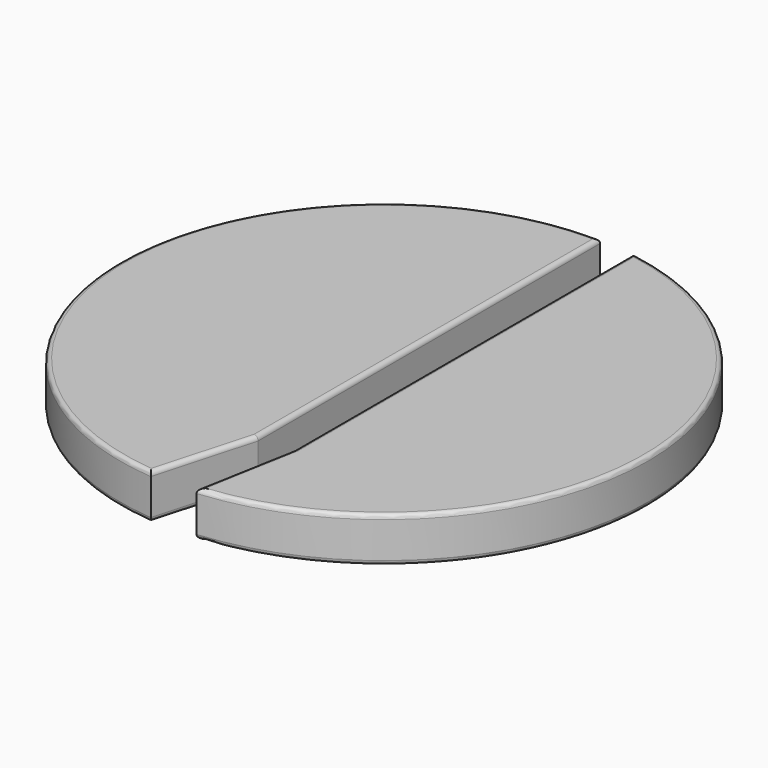
from build123d import *

# Parameters (mm, degrees)
F1_DEPTH      = 3.78
F2_T4_DEPTH   = 40.3204423055
F2_T9_DEPTH   = 12.9439682299
F2_T14_DEPTH  = 12.9439682299
F2_T19_DEPTH  = 40.3204423055
F2_T22_ANGLE  = 177.5138742153
F2_T24_ANGLE  = 177.5138742153
F2_T29_DEPTH  = 40.3204423055
F2_T33_DEPTH  = 12.9439682299
F2_T40_DEPTH  = 40.3204423055
F2_T44_DEPTH  = 12.9439682299
F2_2_T1_DEPTH = 38.6518237684
F2_2_T3_DEPTH = 11.2008796601
F2_2_T6_ANGLE = 180.8453878552
F2_2_T8_ANGLE = 180.8453878552


# Not quite as in the source:
# - a fillet or chamfer that OpenCascade refuses, or shapes differently, is made with other operations: its cross-section is extruded or revolved along the edge and cut away or added


with BuildPart() as f1:
    # F0 (on Top) → F1 (new body)
    with BuildSketch(Plane.XY):
        with BuildLine():
            Line((3.4421672434, -13.8472889727), (1.9314982338, -22.2412890717))
            ThreePointArc((1.9314982338, -22.2412890717), (22.3120303803, -0.7608714143), (3.4421672434, 22.0580395699))
            Line((3.4421672434, 22.0580395699), (3.4421672434, -13.8472889727))
        make_face()
    extrude(amount=F1_DEPTH)

    # F2: fillet of radius 0.3679261469 on 6 edges, made by hand


with BuildPart() as f1b:
    # F0 (on Top) → F1, piece 2 (new body)
    with BuildSketch(Plane.XY):
        with BuildLine():
            Line((0.4208292241, -13.8472889727), (0.4208292241, 22.3210333041))
            ThreePointArc((0.4208292241, 22.3210333041), (-22.2939604848, 1.1768393701), (-1.9314982338, -22.2412890717))
            Line((-1.9314982338, -22.2412890717), (0.4208292241, -13.8472889727))
        make_face()
    extrude(amount=F1_DEPTH)

    # F2#2: fillet of radius 0.3679261469 on 6 edges, made by hand

    # F2_2_s2 → F2_2_t1 (cut)
    with BuildSketch(Plane.XZ.offset(-23.2408486714)):
        with BuildLine():
            ThreePointArc((0.4208292241, 3.4120738531), (0.3130661507, 3.6722369265), (0.0529030772, 3.78))
            Line((0.0529030772, 3.78), (0.4208292241, 3.78))
            Line((0.4208292241, 3.78), (0.4208292241, 3.4120738531))
        make_face()
        with BuildLine():
            ThreePointArc((0.4208292241, 0.3679261469), (0.3130661507, 0.1077630735), (0.0529030772, 0))
            Line((0.0529030772, 0), (0.4208292241, 0))
            Line((0.4208292241, 0), (0.4208292241, 0.3679261469))
        make_face()
    extrude(amount=F2_2_T1_DEPTH, mode=Mode.SUBTRACT)

    # F2_2_s4 → F2_2_t3 (cut)
    with BuildSketch(Plane(origin=(-6.1678788932, -22.0093405225, 0), x_dir=(0, 0, 1), z_dir=(0.2698434566, 0.9629042055, 0))):
        with BuildLine():
            ThreePointArc((3.4120738531, 4.1418185513), (3.6722369265, 4.0340554778), (3.78, 3.7738924044))
            Line((3.78, 3.7738924044), (3.78, 4.1418185513))
            Line((3.78, 4.1418185513), (3.4120738531, 4.1418185513))
        make_face()
        with BuildLine():
            ThreePointArc((0.3679261469, 4.1418185513), (0.1077630735, 4.0340554778), (0, 3.7738924044))
            Line((0, 3.7738924044), (0, 4.1418185513))
            Line((0, 4.1418185513), (0.3679261469, 4.1418185513))
        make_face()
    extrude(amount=F2_2_T3_DEPTH, mode=Mode.SUBTRACT)

    # F2_2_s5 → F2_2_t6 (revolve, cut)
    with BuildSketch(Plane(origin=(0, 0, 0), x_dir=(0, 0, 1), z_dir=(0.9981935886, -0.0600796118, 0))):
        with BuildLine():
            ThreePointArc((3.4120738531, -22.325), (3.6722369265, -22.2172369265), (3.78, -21.9570738531))
            Line((3.78, -21.9570738531), (3.78, -22.325))
            Line((3.78, -22.325), (3.4120738531, -22.325))
        make_face()
    revolve(axis=Axis((0, 0, 3.78), (0, 0, 1)), revolution_arc=F2_2_T6_ANGLE, mode=Mode.SUBTRACT)

    # F2_2_s7 → F2_2_t8 (revolve, cut)
    with BuildSketch(Plane(origin=(0, 0, 0), x_dir=(0, 0, 1), z_dir=(0.9981935886, -0.0600796118, 0))):
        with BuildLine():
            ThreePointArc((0.3679261469, -22.325), (0.1077630735, -22.2172369265), (0, -21.9570738531))
            Line((0, -21.9570738531), (0, -22.325))
            Line((0, -22.325), (0.3679261469, -22.325))
        make_face()
    revolve(axis=Axis((0, 0, 0), (0, 0, 1)), revolution_arc=F2_2_T8_ANGLE, mode=Mode.SUBTRACT)


with BuildPart() as f2_tool2:
    # F2_s3 → F2_t4 (new body)
    with BuildSketch(Plane.XZ.offset(-24.2655964514)):
        with BuildLine():
            ThreePointArc((3.4421672434, 3.4120738531), (3.5499303169, 3.6722369265), (3.8100933903, 3.78))
            Line((3.8100933903, 3.78), (3.8100933903, 3.7873585229))
            Line((3.8100933903, 3.7873585229), (3.4348087205, 3.7873585229))
            Line((3.4348087205, 3.7873585229), (3.4348087205, 3.4120738531))
            Line((3.4348087205, 3.4120738531), (3.4421672434, 3.4120738531))
        make_face()
    extrude(amount=F2_T4_DEPTH)

    split(bisect_by=Plane(origin=(5.7480889705, -1.0344841279, 0), x_dir=(0, 0, 1), z_dir=(-0.9841884548, 0.1771244914, 0)), keep=Keep.TOP)


with BuildPart() as f1_1:
    add(f1.part)

    # F2_t1: cut F2_tool2
    add(f2_tool2.part, mode=Mode.SUBTRACT)


with BuildPart() as f2_tool7:
    # F2_s8 → F2_t9 (new body)
    with BuildSketch(Plane(origin=(-1.9149093372, -10.6401528487, 0), x_dir=(0, 0, 1), z_dir=(-0.1771244914, -0.9841884548, 0))):
        with BuildLine():
            ThreePointArc((3.4120738531, -5.8404352769), (3.6722369265, -5.9481983504), (3.78, -6.2083614238))
            Line((3.78, -6.2083614238), (3.7873585229, -6.2083614238))
            Line((3.7873585229, -6.2083614238), (3.7873585229, -5.833076754))
            Line((3.7873585229, -5.833076754), (3.4120738531, -5.833076754))
            Line((3.4120738531, -5.833076754), (3.4120738531, -5.8404352769))
        make_face()
    extrude(amount=F2_T9_DEPTH)

    split(bisect_by=Plane.YZ.offset(3.4421672434), keep=Keep.BOTTOM)


with BuildPart() as f1_2:
    add(f1_1.part)

    # F2_t6: cut F2_tool7
    add(f2_tool7.part, mode=Mode.SUBTRACT)


with BuildPart() as f2_tool12:
    # F2_s13 → F2_t14 (new body)
    with BuildSketch(Plane(origin=(-1.9149093372, -10.6401528487, 0), x_dir=(0, 0, 1), z_dir=(-0.1771244914, -0.9841884548, 0))):
        with BuildLine():
            ThreePointArc((0.3679261469, -5.8404352769), (0.1077630735, -5.9481983504), (0, -6.2083614238))
            Line((0, -6.2083614238), (-0.0073585229, -6.2083614238))
            Line((-0.0073585229, -6.2083614238), (-0.0073585229, -5.833076754))
            Line((-0.0073585229, -5.833076754), (0.3679261469, -5.833076754))
            Line((0.3679261469, -5.833076754), (0.3679261469, -5.8404352769))
        make_face()
    extrude(amount=F2_T14_DEPTH)

    split(bisect_by=Plane.YZ.offset(3.4421672434), keep=Keep.BOTTOM)


with BuildPart() as f1_3:
    add(f1_2.part)

    # F2_t11: cut F2_tool12
    add(f2_tool12.part, mode=Mode.SUBTRACT)


with BuildPart() as f2_tool17:
    # F2_s18 → F2_t19 (new body)
    with BuildSketch(Plane.XZ.offset(-24.2655964514)):
        with BuildLine():
            ThreePointArc((3.4421672434, 0.3679261469), (3.5499303169, 0.1077630735), (3.8100933903, 0))
            Line((3.8100933903, 0), (3.8100933903, -0.0073585229))
            Line((3.8100933903, -0.0073585229), (3.4348087205, -0.0073585229))
            Line((3.4348087205, -0.0073585229), (3.4348087205, 0.3679261469))
            Line((3.4348087205, 0.3679261469), (3.4421672434, 0.3679261469))
        make_face()
    extrude(amount=F2_T19_DEPTH)

    split(bisect_by=Plane(origin=(5.7480889705, -1.0344841279, 0), x_dir=(0, 0, 1), z_dir=(-0.9841884548, 0.1771244914, 0)), keep=Keep.TOP)


with BuildPart() as f1_4:
    add(f1_3.part)

    # F2_t16: cut F2_tool17
    add(f2_tool17.part, mode=Mode.SUBTRACT)

    # F2_s21 → F2_t22 (revolve, cut)
    with BuildSketch(Plane(origin=(0, 0, 0), x_dir=(0, 0, 1), z_dir=(-0.9999232121, 0.0123923302, 0))):
        with BuildLine():
            ThreePointArc((0.3679261469, -22.325), (0.1077630735, -22.2172369265), (0, -21.9570738531))
            Line((0, -21.9570738531), (-0.0073585229, -21.9570738531))
            Line((-0.0073585229, -21.9570738531), (-0.0073585229, -22.3323585229))
            Line((-0.0073585229, -22.3323585229), (0.3679261469, -22.3323585229))
            Line((0.3679261469, -22.3323585229), (0.3679261469, -22.325))
        make_face()
    revolve(axis=Axis((0, 0, 0), (0, 0, 1)), revolution_arc=F2_T22_ANGLE, mode=Mode.SUBTRACT)

    # F2_s23 → F2_t24 (revolve, cut)
    with BuildSketch(Plane(origin=(0, 0, 0), x_dir=(0, 0, 1), z_dir=(-0.9999232121, 0.0123923302, 0))):
        with BuildLine():
            ThreePointArc((3.4120738531, -22.325), (3.6722369265, -22.2172369265), (3.78, -21.9570738531))
            Line((3.78, -21.9570738531), (3.7873585229, -21.9570738531))
            Line((3.7873585229, -21.9570738531), (3.7873585229, -22.3323585229))
            Line((3.7873585229, -22.3323585229), (3.4120738531, -22.3323585229))
            Line((3.4120738531, -22.3323585229), (3.4120738531, -22.325))
        make_face()
    revolve(axis=Axis((0, 0, 3.78), (0, 0, 1)), revolution_arc=F2_T24_ANGLE, mode=Mode.SUBTRACT)


with BuildPart() as f2_tool27:
    # F2_s28 → F2_t29 (new body)
    with BuildSketch(Plane.XZ.offset(-24.2655964514)):
        with BuildLine():
            ThreePointArc((3.4421672434, 3.4120738531), (3.5499303169, 3.6722369265), (3.8100933903, 3.78))
            Line((3.8100933903, 3.78), (3.8100933903, 3.7873585229))
            Line((3.8100933903, 3.7873585229), (3.4348087205, 3.7873585229))
            Line((3.4348087205, 3.7873585229), (3.4348087205, 3.4120738531))
            Line((3.4348087205, 3.4120738531), (3.4421672434, 3.4120738531))
        make_face()
    extrude(amount=F2_T29_DEPTH)

    split(bisect_by=Plane(origin=(5.7480889705, -1.0344841279, 0), x_dir=(0, 0, 1), z_dir=(0.9841884548, -0.1771244914, 0)), keep=Keep.TOP)


with BuildPart() as f2_tool31:
    # F2_s32 → F2_t33 (new body)
    with BuildSketch(Plane(origin=(-1.9149093372, -10.6401528487, 0), x_dir=(0, 0, 1), z_dir=(-0.1771244914, -0.9841884548, 0))):
        with BuildLine():
            ThreePointArc((3.4120738531, -5.8404352769), (3.6722369265, -5.9481983504), (3.78, -6.2083614238))
            Line((3.78, -6.2083614238), (3.7873585229, -6.2083614238))
            Line((3.7873585229, -6.2083614238), (3.7873585229, -5.833076754))
            Line((3.7873585229, -5.833076754), (3.4120738531, -5.833076754))
            Line((3.4120738531, -5.833076754), (3.4120738531, -5.8404352769))
        make_face()
    extrude(amount=F2_T33_DEPTH)

    split(bisect_by=Plane.YZ.offset(3.4421672434), keep=Keep.TOP)


with BuildPart() as f2_tool27_1:
    add(f2_tool27.part)

    # F2_t35: intersect F2_tool31
    add(f2_tool31.part, mode=Mode.INTERSECT)


with BuildPart() as f1_5:
    add(f1_4.part)

    # F2_t25: cut F2_tool27
    add(f2_tool27_1.part, mode=Mode.SUBTRACT)


with BuildPart() as f2_tool38:
    # F2_s39 → F2_t40 (new body)
    with BuildSketch(Plane.XZ.offset(-24.2655964514)):
        with BuildLine():
            ThreePointArc((3.4421672434, 0.3679261469), (3.5499303169, 0.1077630735), (3.8100933903, 0))
            Line((3.8100933903, 0), (3.8100933903, -0.0073585229))
            Line((3.8100933903, -0.0073585229), (3.4348087205, -0.0073585229))
            Line((3.4348087205, -0.0073585229), (3.4348087205, 0.3679261469))
            Line((3.4348087205, 0.3679261469), (3.4421672434, 0.3679261469))
        make_face()
    extrude(amount=F2_T40_DEPTH)

    split(bisect_by=Plane(origin=(5.7480889705, -1.0344841279, 0), x_dir=(0, 0, 1), z_dir=(0.9841884548, -0.1771244914, 0)), keep=Keep.TOP)


with BuildPart() as f2_tool42:
    # F2_s43 → F2_t44 (new body)
    with BuildSketch(Plane(origin=(-1.9149093372, -10.6401528487, 0), x_dir=(0, 0, 1), z_dir=(-0.1771244914, -0.9841884548, 0))):
        with BuildLine():
            ThreePointArc((0.3679261469, -5.8404352769), (0.1077630735, -5.9481983504), (0, -6.2083614238))
            Line((0, -6.2083614238), (-0.0073585229, -6.2083614238))
            Line((-0.0073585229, -6.2083614238), (-0.0073585229, -5.833076754))
            Line((-0.0073585229, -5.833076754), (0.3679261469, -5.833076754))
            Line((0.3679261469, -5.833076754), (0.3679261469, -5.8404352769))
        make_face()
    extrude(amount=F2_T44_DEPTH)

    split(bisect_by=Plane.YZ.offset(3.4421672434), keep=Keep.TOP)


with BuildPart() as f2_tool38_1:
    add(f2_tool38.part)

    # F2_t46: intersect F2_tool42
    add(f2_tool42.part, mode=Mode.INTERSECT)


with BuildPart() as f1_6:
    add(f1_5.part)

    # F2_t36: cut F2_tool38
    add(f2_tool38_1.part, mode=Mode.SUBTRACT)


solid = Compound([f1b.part, f1_6.part])
